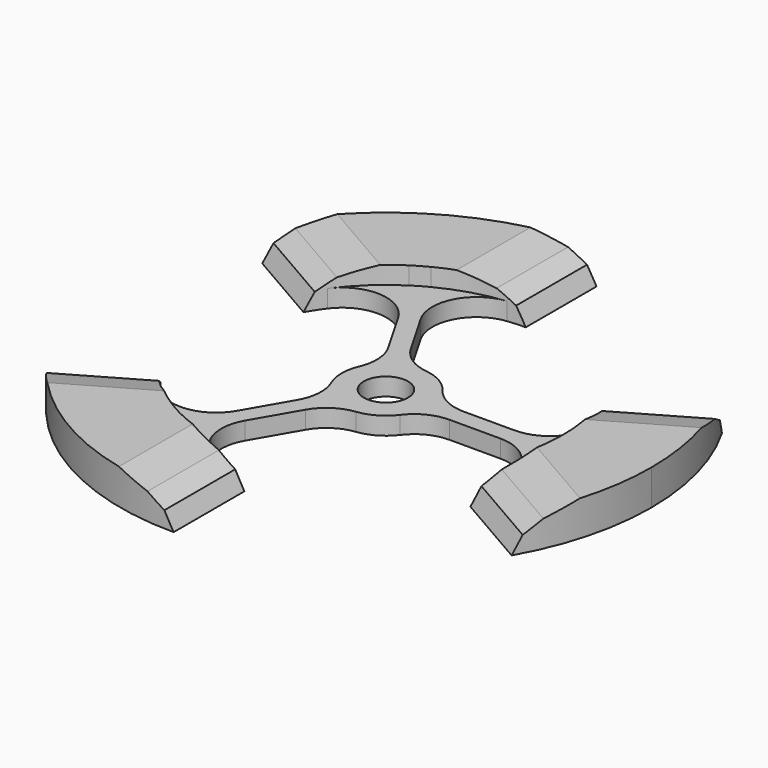
from build123d import *

# Parameters (mm, degrees)
F0_R        = 2.5
F1_DEPTH    = 2
F2_DEPTH    = 4
F3_T1_DEPTH = 2
F4_T1_DEPTH = 32.4048198529
F4_T3_DEPTH = 32.4048198529
F4_T5_DEPTH = 32.4048198529
F5_SIZE2    = 2.309391
F5_SIZE     = 3.99999
F5_2_SIZE2  = 2.309391
F5_2_SIZE   = 3.99999
F5_3_SIZE2  = 2.309391
F5_3_SIZE   = 3.99999
F6_SIZE     = 2.5
F7_SIZE     = 2


# Not quite as in the source:
# - a fillet or chamfer that OpenCascade refuses, or shapes differently, is made with other operations: its cross-section is extruded or revolved along the edge and cut away or added
# - a fillet or chamfer is up to 0.001 mm smaller than in the source, because OpenCascade refuses the exact size


with BuildPart() as f1:
    # F0 (on Top) → F1 (new body)
    with BuildSketch(Plane.XY):
        with BuildLine():
            ThreePointArc((-10.8535175815, -16.798843892), (-10, -17.3205080757), (-9.1214667739, -17.798843892))
            Line((-9.1214667739, -17.798843892), (-1.583464339, -4.7426406871))
            ThreePointArc((-1.583464339, -4.7426406871), (-2.5, -4.3301270189), (-3.3155151466, -3.7426406871))
            Line((-3.3155151466, -3.7426406871), (-10.8535175815, -16.798843892))
        make_face()
        with BuildLine():
            Line((-1.583464339, 4.7426406871), (-9.1214667739, 17.798843892))
            ThreePointArc((-9.1214667739, 17.798843892), (-10, 17.3205080757), (-10.8535175815, 16.798843892))
            Line((-10.8535175815, 16.798843892), (-3.3155151466, 3.7426406871))
            ThreePointArc((-3.3155151466, 3.7426406871), (-2.5, 4.3301270189), (-1.583464339, 4.7426406871))
        make_face()
        with BuildLine():
            ThreePointArc((20, 0), (19.9937451108, 0.5001564212), (19.9749843554, 1))
            Line((19.9749843554, 1), (4.8989794856, 1))
            ThreePointArc((4.8989794856, 1), (4.974680765, 0.50254481), (5, 0))
            ThreePointArc((5, 0), (4.974680765, -0.50254481), (4.8989794856, -1))
            Line((4.8989794856, -1), (19.9749843554, -1))
            ThreePointArc((19.9749843554, -1), (19.9937451108, -0.5001564212), (20, 0))
        make_face()
        with BuildLine():
            ThreePointArc((5, 0), (4.974680765, 0.50254481), (4.8989794856, 1))
            ThreePointArc((4.8989794856, 1), (2.5, 4.3301270189), (-1.583464339, 4.7426406871))
            ThreePointArc((-1.583464339, 4.7426406871), (-2.5, 4.3301270189), (-3.3155151466, 3.7426406871))
            ThreePointArc((-3.3155151466, 3.7426406871), (-5, 0), (-3.3155151466, -3.7426406871))
            ThreePointArc((-3.3155151466, -3.7426406871), (-2.5, -4.3301270189), (-1.583464339, -4.7426406871))
            ThreePointArc((-1.583464339, -4.7426406871), (2.5, -4.3301270189), (4.8989794856, -1))
            ThreePointArc((4.8989794856, -1), (4.974680765, -0.50254481), (5, 0))
        make_face()
        Circle(F0_R, mode=Mode.SUBTRACT)
    extrude(amount=F1_DEPTH)

    # F0 (on Top) → F2 (join)
    with BuildSketch(Plane.XY):
        with BuildLine():
            Line((0, 20), (0, 30))
            ThreePointArc((0, 30), (-15, 25.9807621135), (-25.9807621135, 15))
            Line((-25.9807621135, 15), (-17.3205080757, 10))
            ThreePointArc((-17.3205080757, 10), (-14.4913767462, 13.7840487521), (-10.8535175815, 16.798843892))
            ThreePointArc((-10.8535175815, 16.798843892), (-10, 17.3205080757), (-9.1214667739, 17.798843892))
            ThreePointArc((-9.1214667739, 17.798843892), (-4.6916480132, 19.4419247741), (0, 20))
        make_face()
        with BuildLine():
            ThreePointArc((25.9807621135, -15), (28.9777747887, -7.7645713531), (30, 0))
            ThreePointArc((30, 0), (28.9777747887, 7.7645713531), (25.9807621135, 15))
            Line((25.9807621135, 15), (17.3205080757, 10))
            ThreePointArc((17.3205080757, 10), (19.1830247594, 5.657876022), (19.9749843554, 1))
            ThreePointArc((19.9749843554, 1), (19.9937451108, 0.5001564212), (20, 0))
            ThreePointArc((20, 0), (19.9937451108, -0.5001564212), (19.9749843554, -1))
            ThreePointArc((19.9749843554, -1), (19.1830247594, -5.657876022), (17.3205080757, -10))
            Line((17.3205080757, -10), (25.9807621135, -15))
        make_face()
        with BuildLine():
            ThreePointArc((-25.9807621135, -15), (-15, -25.9807621135), (0, -30))
            Line((0, -30), (0, -20))
            ThreePointArc((0, -20), (-4.6916480132, -19.4419247741), (-9.1214667739, -17.798843892))
            ThreePointArc((-9.1214667739, -17.798843892), (-10, -17.3205080757), (-10.8535175815, -16.798843892))
            ThreePointArc((-10.8535175815, -16.798843892), (-14.4913767462, -13.7840487521), (-17.3205080757, -10))
            Line((-17.3205080757, -10), (-25.9807621135, -15))
        make_face()
    extrude(amount=F2_DEPTH)

    # F3: fillet of radius 5 on 12 edges, made by hand

    # F3_s2 → F3_t1 (join)
    with BuildSketch(Plane.XY):
        with BuildLine():
            ThreePointArc((-2.2369481596, 19.8745078664), (-6.1410694312, 17.1594186926), (-6.0078381387, 12.4058808998))
            Line((-6.0078381387, 12.4058808998), (-9.1214667739, 17.798843892))
            ThreePointArc((-9.1214667739, 17.798843892), (-5.7732566792, 19.148616329), (-2.2369481596, 19.8745078664))
        make_face()
        with BuildLine():
            ThreePointArc((-16.0933546202, 11.8745078664), (-11.7899577863, 13.8980314801), (-7.7398889462, 11.4058808998))
            Line((-7.7398889462, 11.4058808998), (-10.8535175815, 16.798843892))
            ThreePointArc((-10.8535175815, 16.798843892), (-13.6965598486, 14.5740951113), (-16.0933546202, 11.8745078664))
        make_face()
        with BuildLine():
            ThreePointArc((18.3303027798, 8), (17.9310272175, 3.2613872125), (13.7477270849, 1))
            Line((13.7477270849, 1), (19.9749843554, 1))
            ThreePointArc((19.9749843554, 1), (19.4698165279, 4.5745212177), (18.3303027798, 8))
        make_face()
        with BuildLine():
            ThreePointArc((13.7477270849, -1), (17.9310272175, -3.2613872125), (18.3303027798, -8))
            ThreePointArc((18.3303027798, -8), (19.4698165279, -4.5745212177), (19.9749843554, -1))
            Line((19.9749843554, -1), (13.7477270849, -1))
        make_face()
        with BuildLine():
            ThreePointArc((-16.0933546202, -11.8745078664), (-11.7899577863, -13.8980314801), (-7.7398889462, -11.4058808998))
            Line((-7.7398889462, -11.4058808998), (-10.8535175815, -16.798843892))
            ThreePointArc((-10.8535175815, -16.798843892), (-13.6965598486, -14.5740951113), (-16.0933546202, -11.8745078664))
        make_face()
        with BuildLine():
            ThreePointArc((-2.2369481596, -19.8745078664), (-6.1410694312, -17.1594186926), (-6.0078381387, -12.4058808998))
            Line((-6.0078381387, -12.4058808998), (-9.1214667739, -17.798843892))
            ThreePointArc((-9.1214667739, -17.798843892), (-5.7732566792, -19.148616329), (-2.2369481596, -19.8745078664))
        make_face()
        with BuildLine():
            ThreePointArc((-3.1339745962, 7.4282032303), (-1.5587969348, 5.7556435797), (0.5980762114, 4.9641016151))
            ThreePointArc((0.5980762114, 4.9641016151), (-0.5049838375, 4.9744337692), (-1.583464339, 4.7426406871))
            Line((-1.583464339, 4.7426406871), (-3.1339745962, 7.4282032303))
        make_face()
        with BuildLine():
            ThreePointArc((8, 1), (5.7639320225, 1.527864045), (4, 3))
            ThreePointArc((4, 3), (4.5604779323, 2.0498880528), (4.8989794856, 1))
            Line((4.8989794856, 1), (8, 1))
        make_face()
        with BuildLine():
            ThreePointArc((-4.8660254038, 6.4282032303), (-4.2051350877, 4.2277795347), (-4.5980762114, 1.9641016151))
            ThreePointArc((-4.5980762114, 1.9641016151), (-4.0554940948, 2.9245457164), (-3.3155151466, 3.7426406871))
            Line((-3.3155151466, 3.7426406871), (-4.8660254038, 6.4282032303))
        make_face()
        with BuildLine():
            ThreePointArc((-4.5980762114, -1.9641016151), (-4.2051350877, -4.2277795347), (-4.8660254038, -6.4282032303))
            Line((-4.8660254038, -6.4282032303), (-3.3155151466, -3.7426406871))
            ThreePointArc((-3.3155151466, -3.7426406871), (-4.0554940948, -2.9245457164), (-4.5980762114, -1.9641016151))
        make_face()
        with BuildLine():
            ThreePointArc((-3.1339745962, -7.4282032303), (-1.5587969348, -5.7556435797), (0.5980762114, -4.9641016151))
            ThreePointArc((0.5980762114, -4.9641016151), (-0.5049838375, -4.9744337692), (-1.583464339, -4.7426406871))
            Line((-1.583464339, -4.7426406871), (-3.1339745962, -7.4282032303))
        make_face()
        with BuildLine():
            ThreePointArc((4, -3), (5.7639320225, -1.527864045), (8, -1))
            Line((8, -1), (4.8989794856, -1))
            ThreePointArc((4.8989794856, -1), (4.5604779323, -2.0498880528), (4, -3))
        make_face()
    extrude(amount=F3_T1_DEPTH)

    # F4: chamfer of 2.5 x 4.3301270189 on 3 edges, made by hand

    # F4_s2 → F4_t1 (cut)
    with BuildSketch(Plane(origin=(-7.6189364958, -4.3987950368, 0), x_dir=(0, 0, 1), z_dir=(-0.8660254038, -0.5, 0))):
        Polygon((-0.3301270189, 0), (4, -2.5), (4, 0), align=None)
    extrude(amount=F4_T1_DEPTH, mode=Mode.SUBTRACT)

    # F4_s4 → F4_t3 (cut)
    with BuildSketch(Plane.XZ.offset(-41.2024099265)):
        Polygon((-2.5, 4), (0, -0.3301270189), (0, 4), align=None)
    extrude(amount=F4_T3_DEPTH, mode=Mode.SUBTRACT)

    # F4_s6 → F4_t5 (cut)
    with BuildSketch(Plane(origin=(7.6189364958, -4.3987950368, 0), x_dir=(0, 0, 1), z_dir=(0.8660254038, -0.5, 0))):
        Polygon((-0.3301270189, 0), (4, -2.5), (4, 0), align=None)
    extrude(amount=F4_T5_DEPTH, mode=Mode.SUBTRACT)

    # F5 (size 4 and 2.3094010768 in the source; OpenCascade refuses exactly that, so slightly less here)
    f5_edges = [f1.edges().sort_by_distance(p)[0] for p in [
        (21.650635, 12.5, 4),
    ]]
    f5_side = f1.faces().sort_by_distance((21.650635, 12.5, 2))[0]
    chamfer(f5_edges, length=F5_SIZE, length2=F5_SIZE2, reference=f5_side)

    # F5#2 (size 4 and 2.3094010768 in the source; OpenCascade refuses exactly that, so slightly less here)
    f5_2_edges = [f1.edges().sort_by_distance(p)[0] for p in [
        (-21.650635, 12.5, 4),
    ]]
    f5_2_side = f1.faces().sort_by_distance((-21.650635, 12.5, 2))[0]
    chamfer(f5_2_edges, length=F5_2_SIZE, length2=F5_2_SIZE2, reference=f5_2_side)

    # F5#3 (size 4 and 2.3094010768 in the source; OpenCascade refuses exactly that, so slightly less here)
    f5_3_edges = [f1.edges().sort_by_distance(p)[0] for p in [
        (0, -25, 4),
    ]]
    f5_3_side = f1.faces().sort_by_distance((0, -25, 2))[0]
    chamfer(f5_3_edges, length=F5_3_SIZE, length2=F5_3_SIZE2, reference=f5_3_side)

    # F6
    f6_edges = [f1.edges().sort_by_distance(p)[0] for p in [
        (-20.399464, 14.444291, 4),
        (-2.5, 24.869393, 4),
        (22.708855, 10.444309, 4),
        (22.787526, -10.269633, 4),
        (-2.309391, -24.8886, 4),
        (-20.287526, -14.59976, 4),
    ]]
    chamfer(f6_edges, length=F6_SIZE)

    # F7
    f7_edges = [f1.edges().sort_by_distance(p)[0] for p in [
        (-5, 24.472658, 4),
        (-18.823804, 16.421335, 4),
        (23.633195, 8.091225, 4),
        (23.693943, -7.906202, 4),
        (-4.809391, -24.51256, 4),
        (-18.693943, -16.566456, 4),
    ]]
    chamfer(f7_edges, length=F7_SIZE)


solid = f1.part
